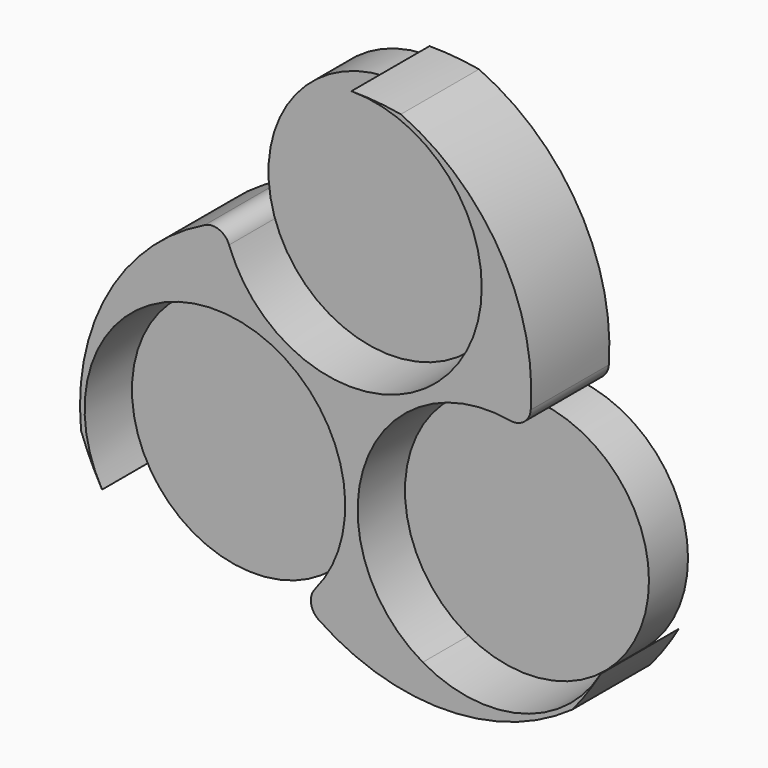
from build123d import *

# Parameters (mm, degrees)
F0_R            = 29.5
F1_DEPTH        = 10
F3_DEPTH        = 10.001
F3_COPIES_COUNT = 3
F4_R            = 1.8
F5_R            = 12.5
F6_DEPTH        = 5
F6_COPIES_COUNT = 3


# Not quite as in the source:
# - a feature of the source that left no trace in its solid (it failed there, or was rolled back) is left out
# - a pattern or mirror of a feature is missing from the dataset's text; its kind, count and spacing are read off the source's solid


with BuildPart() as f1:
    # F0 (on Front) → F1 (new body)
    with BuildSketch(Plane.XZ):
        Circle(F0_R)
    extrude(amount=F1_DEPTH)

    # F2 (on face) → F3 (cut, through all)
    with BuildSketch(Plane.XZ.offset(10)):
        with BuildLine():
            ThreePointArc((5.19e-08, 29.5), (-10.3715819967, 24.555854269), (-13.0613006149, 13.3853706199))
            ThreePointArc((-13.0613006149, 13.3853706199), (1.3895790428, 2.8713808608), (13.3505662359, 16.1494337641))
            ThreePointArc((13.3505662359, 16.1494337641), (9.4402759364, 25.5897096638), (5.19e-08, 29.5))
        make_face()
        with BuildLine():
            ThreePointArc((-27.7019032287, -10.1417235966), (-24.3788882915, 4.10928247), (-13.0613006149, 13.3853706199))
            ThreePointArc((-13.0613006149, 13.3853706199), (-10.3715819967, 24.555854269), (5.19e-08, 29.5))
            ThreePointArc((5.19e-08, 29.5), (-24.18088961, 16.8977684227), (-27.7019032287, -10.1417235966))
        make_face()
    f3 = extrude(amount=-F3_DEPTH, mode=Mode.SUBTRACT)

    # F3_copies: F3 ×3 about axis
    f3_copies_axis = Axis((0, 0, 0), (0, 1, 0))
    for i in range(1, F3_COPIES_COUNT):
        add(f3.rotate(f3_copies_axis, i * 360 / F3_COPIES_COUNT), mode=Mode.SUBTRACT)

    # F4
    f4_edges = [f1.edges().sort_by_distance(p)[0] for p in [
        (-13.061301, -5, 13.385371),
        (-5.061421, -5, -18.004103),
        (18.122721, -5, 4.618733),
    ]]
    fillet(f4_edges, radius=F4_R)


with BuildPart() as f6:
    # F5 (on Front) → F6 (new body)
    with BuildSketch(Plane.XZ):
        with Locations((-13.9858198965, -8.0747168821)):
            Circle(F5_R)
    extrude(amount=F6_DEPTH)


with BuildPart() as f6_copies_1:
    # F6_copies: instance of F6
    add(f6.part.rotate(Axis((0, 0, 0), (0, 1, 0)), 1 * 360 / F6_COPIES_COUNT))


with BuildPart() as f6_copies_2:
    # F6_copies: instance of F6
    add(f6.part.rotate(Axis((0, 0, 0), (0, 1, 0)), 2 * 360 / F6_COPIES_COUNT))


solid = Compound([f1.part, f6.part, f6_copies_1.part, f6_copies_2.part])
